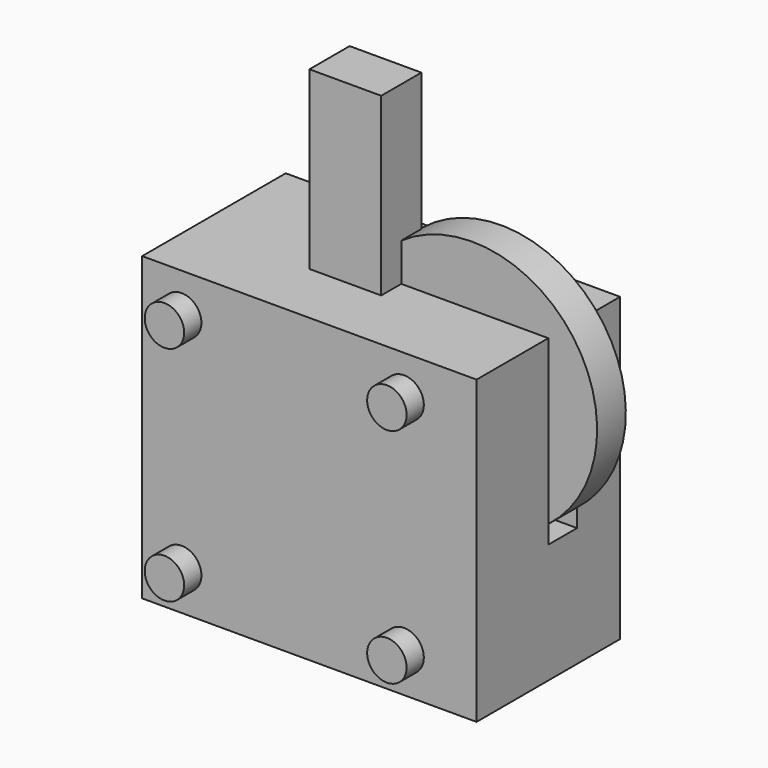
from build123d import *

# Parameters (mm, degrees)
F0_W      = 42
F0_H      = 42
F1_DEPTH  = 12.5
F2_R      = 1.5
F3_DEPTH  = 25.001
F6_R      = 17.4
F7_DEPTH  = 5
F8_DEPTH  = 4.6
F9_W      = 10
F9_H      = 7
F10_DEPTH = 24.5
F11_R     = 2.75
F12_DEPTH = 3


with BuildPart() as f1:
    # F0 (on Front) → F1 (new body, symmetric)
    with BuildSketch(Plane.XZ):
        Rectangle(F0_W, F0_H)
    extrude(amount=F1_DEPTH, both=True)

    # F2 (on face) → F3 (cut, through all)
    with BuildSketch(Plane.XZ.offset(12.5)):
        with Locations((-15.5, 15.5)):
            Circle(F2_R)
        with Locations((15.5, 15.5)):
            Circle(F2_R)
        with Locations((-15.5, -15.5)):
            Circle(F2_R)
        with Locations((15.5, -15.5)):
            Circle(F2_R)
    extrude(amount=-F3_DEPTH, mode=Mode.SUBTRACT)

    # F4 (on Front) → F5 (revolve, cut)
    with BuildSketch(Plane.XZ):
        Polygon((13.55, -8.3), (5.55, -8.3), (5.55, -21), (13.55, -21), (13.55, -18), (11.55, -18), (11.55, -12), (13.55, -12), align=None)
    revolve(axis=Axis((5.55, 0, -42.7623434187), (0, 0, -1)), mode=Mode.SUBTRACT)

    # F6 (on Front) → F7 (join)
    with BuildSketch(Plane.XZ):
        with Locations((15, 12)):
            Circle(F6_R)
    extrude(amount=-F7_DEPTH)

    # F8 (add): a face of the model
    f8_faces = [f1.faces().sort_by_distance(p)[0] for p in [
        (21, -0.3429519104, -1.1432103634),
    ]]
    extrude(f8_faces, amount=F8_DEPTH)

    # F9 (on face) → F10 (join)
    with BuildSketch(Plane.XY.offset(21)):
        with Locations((0.1083916248, 0)):
            Rectangle(F9_W, F9_H)
    extrude(amount=F10_DEPTH)

    # F11 (on face) → F12 (join)
    with BuildSketch(Plane.XZ.offset(12.5)):
        with Locations((-15.5, 15.5)):
            Circle(F11_R)
        with Locations((-15.5, -15.5)):
            Circle(F11_R)
        with Locations((15.5, -15.5)):
            Circle(F11_R)
        with Locations((15.5, 15.5)):
            Circle(F11_R)
    extrude(amount=F12_DEPTH)


solid = f1.part
